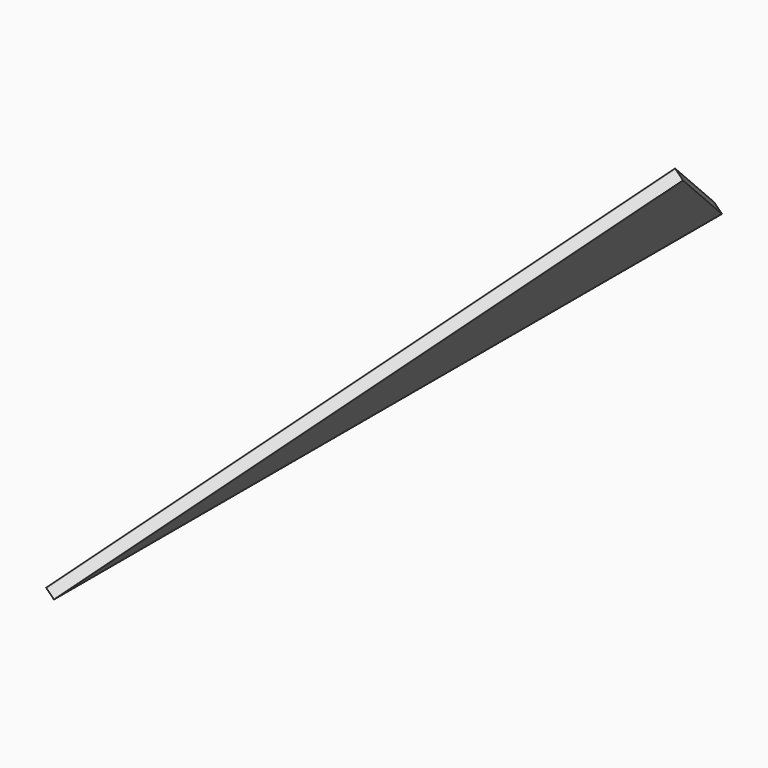
from build123d import *

# Parameters (mm, degrees)
F2_DEPTH = 2
F3_ANGLE = 45


# Not quite as in the source:
# - a feature of the source that left no trace in its solid (it failed there, or was rolled back) is left out


with BuildPart() as f2:
    # F0 (on Top) → F2 (new body)
    with BuildSketch(Plane.XY):
        Polygon((0, 0), (-75.4753425717, 75.4709467292), (-75.4753425717, -74.6340751648), align=None)
    extrude(amount=F2_DEPTH)


with BuildPart() as f2_1:
    # F3: moved
    add(f2.part.rotate(Axis((-75.4753425717, 0.4184357822, 0), (0, -1, 0)), F3_ANGLE))


solid = f2_1.part
